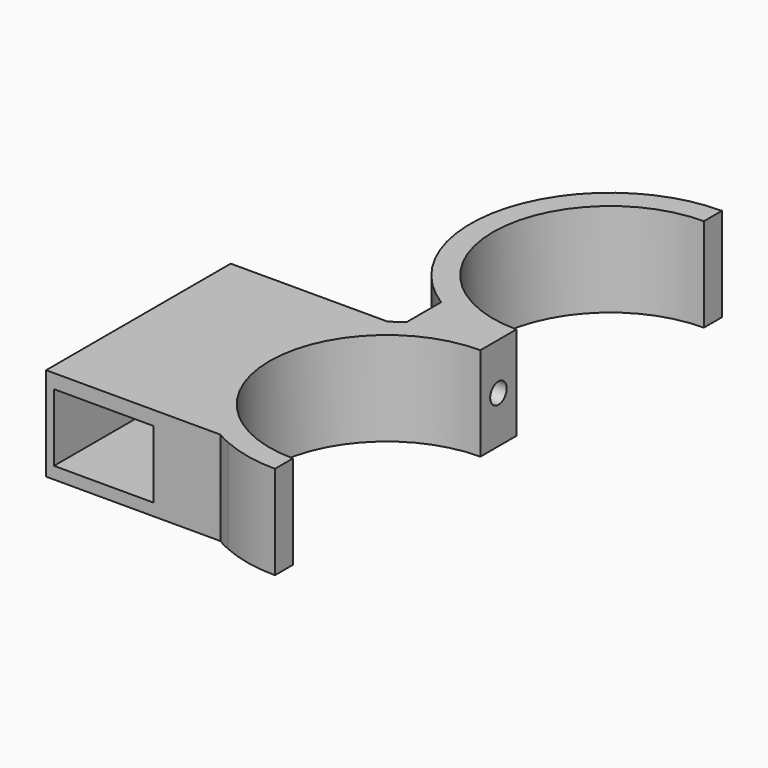
from build123d import *

# Parameters (mm, degrees)
F1_DEPTH = 25
F2_R     = 2.75
F3_DEPTH = 19.9132636974
F4_R     = 5
F5_DEPTH = 2
F6_DEPTH = 25
F7_W     = 26.5
F7_H     = 18
F8_DEPTH = 61.5532770753


with BuildPart() as f1:
    # F0 (on Top) → F1 (new body)
    with BuildSketch(Plane.XY):
        with BuildLine():
            Line((0, 68.5), (0, 74.5))
            ThreePointArc((0, 74.5), (-35.7787380635, 47.6155391844), (-19.9122636974, 5.7688269843))
            ThreePointArc((-19.9122636974, 5.7688269843), (-10.3655391695, 1.4712619322), (3.09e-08, 0))
            Line((0, 0), (0, 6))
            ThreePointArc((0, 6), (-31.25, 37.25), (0, 68.5))
        make_face()
        with BuildLine():
            ThreePointArc((3.09e-08, 0), (-10.3655391695, 1.4712619322), (-19.9122636974, 5.7688269843))
            Line((-19.9122636974, 5.7688269843), (-19.9122636974, -5.7688269843))
            ThreePointArc((-19.9122636974, -5.7688269843), (-17.5050379591, -4.3693651818), (-15, -3.1536292254))
            ThreePointArc((-15, -3.1536292254), (-7.6639639933, -0.7969321468), (3.09e-08, 0))
        make_face()
        with BuildLine():
            Line((0, -6), (0, 0))
            ThreePointArc((3.09e-08, 0), (-7.6639639933, -0.7969321468), (-15, -3.1536292254))
            Line((-15, -3.1536292254), (-15, -8.0031603575))
            Line((-15, -8.0031603575), (-23.0691324268, -8.0031603575))
            ThreePointArc((-23.0691324268, -8.0031603575), (-27.5276929828, -12.1544103666), (-31.25, -16.9768650673))
            ThreePointArc((-31.25, -16.9768650673), (-37.25, -37.25), (-31.25, -57.5231349327))
            ThreePointArc((-31.25, -57.5231349327), (-25.6133761152, -64.2965795246), (-18.543370794, -69.5564374328))
            Line((-18.543370794, -69.5564374328), (-15, -69.5564374328))
            Line((-15, -69.5564374328), (-15, -71.3463707746))
            ThreePointArc((-15, -71.3463707746), (-7.6639640084, -73.70306785), (0, -74.5))
            Line((0, -74.5), (0, -68.5))
            ThreePointArc((0, -68.5), (-31.25, -37.25), (0, -6))
        make_face()
        with BuildLine():
            ThreePointArc((-18.543370794, -69.5564374328), (-16.7955469217, -70.4986406279), (-15, -71.3463707746))
            Line((-15, -71.3463707746), (-15, -69.5564374328))
            Line((-15, -69.5564374328), (-18.543370794, -69.5564374328))
        make_face()
    extrude(amount=F1_DEPTH)

    # F2 (on face) → F3 (cut, through all)
    with BuildSketch(Plane(origin=(-19.9122636974, 0, 0), x_dir=(0, -1, 0), z_dir=(-1, 0, 0))):
        with Locations((0, 12.5)):
            Circle(F2_R)
    extrude(amount=-F3_DEPTH, mode=Mode.SUBTRACT)

    # F4 (on face) → F5 (cut)
    with BuildSketch(Plane(origin=(-19.9122636974, 0, 0), x_dir=(0, -1, 0), z_dir=(-1, 0, 0))):
        with Locations((0, 12.5)):
            Circle(F4_R)
    extrude(amount=-F5_DEPTH, mode=Mode.SUBTRACT)

    # F0 (on Top) → F6 (join)
    with BuildSketch(Plane.XY):
        with BuildLine():
            ThreePointArc((-31.25, -57.5231349327), (-37.25, -37.25), (-31.25, -16.9768650673))
            Line((-31.25, -16.9768650673), (-31.25, -12.7797988951))
            Line((-31.25, -12.7797988951), (-48.75, -12.7797988951))
            Line((-48.75, -12.7797988951), (-48.75, -64.7797988951))
            Line((-48.75, -64.7797988951), (-31.25, -64.7797988951))
            Line((-31.25, -64.7797988951), (-31.25, -57.5231349327))
        make_face()
        with BuildLine():
            ThreePointArc((-31.25, -16.9768650673), (-27.5276929828, -12.1544103666), (-23.0691324268, -8.0031603575))
            Line((-23.0691324268, -8.0031603575), (-65, -8.0031603575))
            Line((-65, -8.0031603575), (-65, -69.5564374328))
            Line((-65, -69.5564374328), (-18.543370794, -69.5564374328))
            ThreePointArc((-18.543370794, -69.5564374328), (-25.6133761152, -64.2965795246), (-31.25, -57.5231349327))
            Line((-31.25, -57.5231349327), (-31.25, -64.7797988951))
            Line((-31.25, -64.7797988951), (-48.75, -64.7797988951))
            Line((-48.75, -64.7797988951), (-48.75, -12.7797988951))
            Line((-48.75, -12.7797988951), (-31.25, -12.7797988951))
            Line((-31.25, -12.7797988951), (-31.25, -16.9768650673))
        make_face()
        with BuildLine():
            ThreePointArc((-15, -3.1536292254), (-17.5050379591, -4.3693651818), (-19.9122636974, -5.7688269843))
            ThreePointArc((-19.9122636974, -5.7688269843), (-21.5197157184, -6.8449948956), (-23.0691324268, -8.0031603575))
            Line((-23.0691324268, -8.0031603575), (-15, -8.0031603575))
            Line((-15, -8.0031603575), (-15, -3.1536292254))
        make_face()
    extrude(amount=F6_DEPTH)

    # F7 (on face) → F8 (cut, through all)
    with BuildSketch(Plane.XZ.offset(69.5564374328)):
        with Locations((-49.6350233853, 12.2272316366)):
            Rectangle(F7_W, F7_H)
    extrude(amount=-F8_DEPTH, mode=Mode.SUBTRACT)


solid = f1.part
